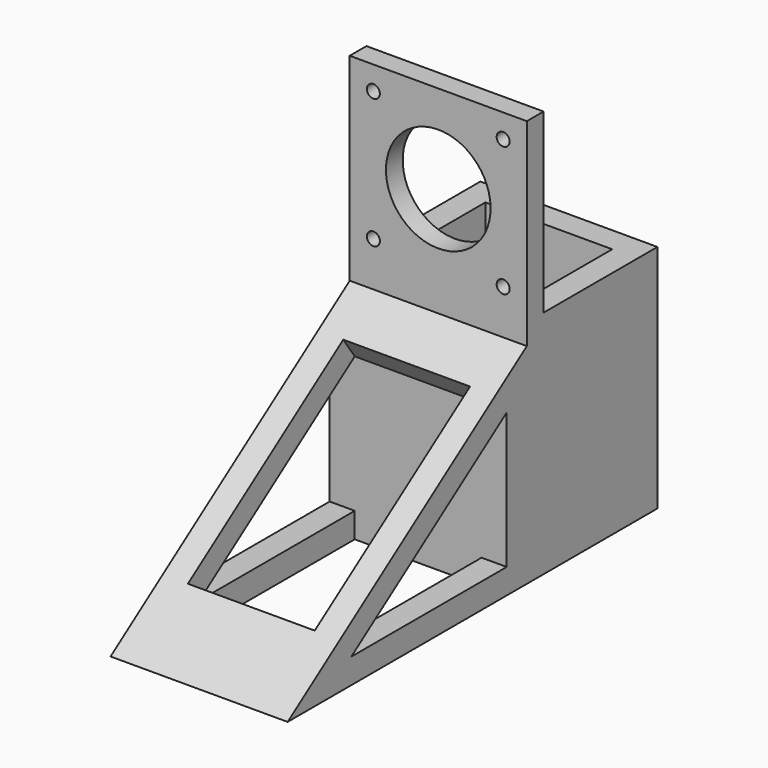
from build123d import *

# Parameters (mm, degrees)
F0_W      = 42.3
F0_H      = 42.3
F0_R      = 12.5
F1_DEPTH  = 5
F2_D      = 3.1
F0_H_2    = 5
F3_DEPTH  = 5
F4_DEPTH  = 34
F5_W      = 30.3
F5_H      = 28
F6_DEPTH  = 5
F7_DEPTH  = 50
F9_DEPTH  = 42.3
F10_W     = 30.3
F10_H     = 56.616878205
F11_DEPTH = 25
F12_W     = 30.3
F12_H     = 46.3778315229
F13_DEPTH = 25


with BuildPart() as f1:
    # F0 (on Front) → F1 (new body)
    with BuildSketch(Plane.XZ):
        Rectangle(F0_W, F0_H)
        Circle(F0_R, mode=Mode.SUBTRACT)
    extrude(amount=F1_DEPTH)

    # F2 (through all)
    with Locations(Plane(origin=(0, 0, 0), x_dir=(1, 0, 0), z_dir=(0, 1, 0))):
        with Locations((-15.5, -15.5), (-15.5, 15.5), (15.5, 15.5), (15.5, -15.5)):
            Hole(F2_D / 2)

    # F0 (on Front) → F3 (join)
    with BuildSketch(Plane.XZ):
        with Locations((0, -23.65)):
            Rectangle(F0_W, F0_H_2)
    extrude(amount=F3_DEPTH)

    # F0 (on Front) → F4 (join)
    with BuildSketch(Plane.XZ):
        with Locations((0, -23.65)):
            Rectangle(F0_W, F0_H_2)
    extrude(amount=-F4_DEPTH)

    # F5 (on face) → F6 (cut)
    with BuildSketch(Plane.XY.offset(-21.15)):
        with Locations((0, 14)):
            Rectangle(F5_W, F5_H)
    extrude(amount=-F6_DEPTH, mode=Mode.SUBTRACT)

    # F7 (add): a face of the model
    f7_faces = [f1.faces().sort_by_distance(p)[0] for p in [
        (0, -4.4246488029, -26.15),
    ]]
    extrude(f7_faces, amount=F7_DEPTH)

    # F8 (on face) → F9 (join)
    with BuildSketch(Plane.YZ.offset(21.15)):
        Polygon((-76.4074003371, -76.15), (-5, -76.15), (-5, -26.15), align=None)
        Polygon((-57.3778315229, -70.15), (-11, -37.6758927618), (-11, -70.15), align=None, mode=Mode.SUBTRACT)
    extrude(amount=-F9_DEPTH)

    # F10 (on face) → F11 (cut)
    with BuildSketch(Plane(origin=(0, 14.0829899932, -20.1125940878), x_dir=(1, 0, 0), z_dir=(0, 0.5735764364, -0.8191520443))):
        with Locations((0, 58.9291158964)):
            Rectangle(F10_W, F10_H)
    extrude(amount=-F11_DEPTH, mode=Mode.SUBTRACT)

    # F12 (on face) → F13 (cut)
    with BuildSketch(Plane.XY.offset(-70.15)):
        with Locations((0, -34.1889157615)):
            Rectangle(F12_W, F12_H)
    extrude(amount=-F13_DEPTH, mode=Mode.SUBTRACT)


solid = f1.part
